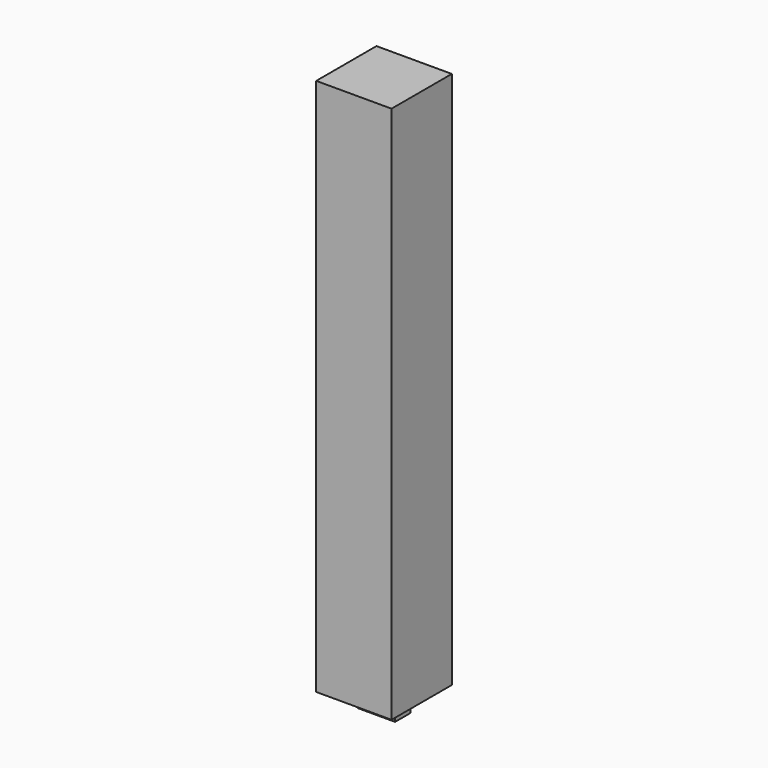
from build123d import *

# Parameters (mm, degrees)
F0_W     = 3.5
F0_H     = 1.8
F1_DEPTH = 1.8
F2_W     = 7
F2_H     = 7
F2_W_2   = 3.5
F2_H_2   = 1.8
F3_DEPTH = 50


# Not quite as in the source:
# - a feature names something its author has since deleted; it is built from what else it names


with BuildPart() as f1:
    # F0 (on Front) → F1 (new body)
    with BuildSketch(Plane.XZ):
        with Locations((0, -25.45)):
            Rectangle(F0_W, F0_H)
    extrude(amount=F1_DEPTH)

    # F2 (on face) → F3 (join)
    with BuildSketch(Plane.XY.offset(-24.55)):
        with Locations((0, -0.9)):
            Rectangle(F2_W, F2_H)
        with Locations((0, -0.9)):
            Rectangle(F2_W_2, F2_H_2, mode=Mode.SUBTRACT)
        with Locations((0, -0.9)):
            Rectangle(F2_W_2, F2_H_2)
    extrude(amount=F3_DEPTH)


solid = f1.part
